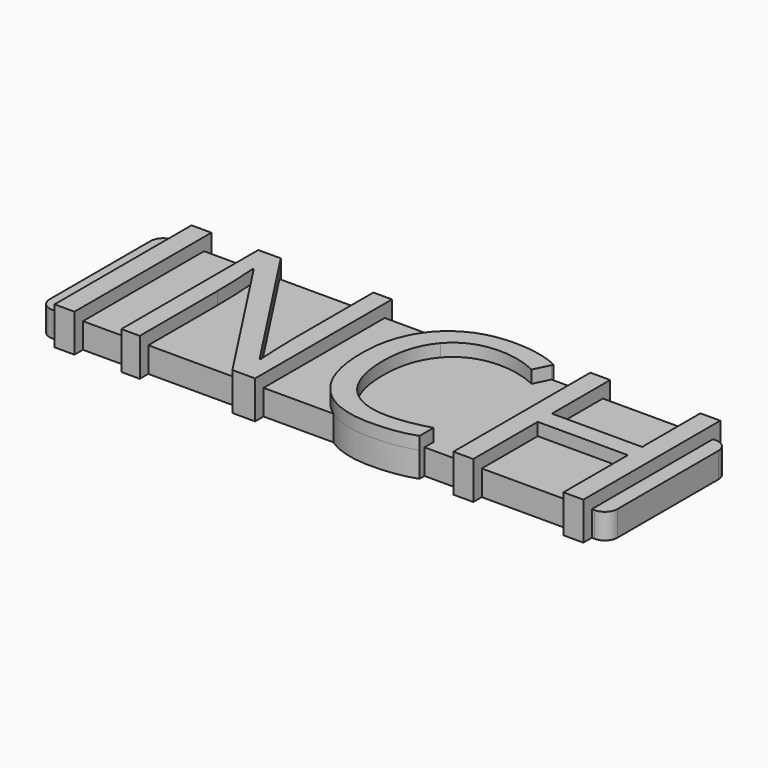
from build123d import *

# Parameters (mm, degrees)
F0_W          = 90
F0_H          = 24
F1_DEPTH      = 4
F2_R          = 2
F3_W          = 3.1525826242
F3_H          = 1.6790025727
F3_H_2        = 1.4474569563
F3_H_3        = 24
F3_W_2        = 2.9150999406
F3_W_3        = 2.9507223432
F4_DEPTH      = 2
F4_DEPTH_BACK = 4
F5_TEXT_SIZE  = 17.3611111111
F6_DEPTH      = 1.5


# Not quite as in the source:
# - a feature names something its author has since deleted; it is built from what else it names
# - Text() gives the source's letters only with a copy of the font that has no kerning and outlines rounded to 1/6400 em; it was checked with that copy


with BuildPart() as f1:
    # F0 (on Top) → F1 (new body)
    with BuildSketch(Plane.XY):
        Rectangle(F0_W, F0_H)
    extrude(amount=F1_DEPTH)

    # F2
    f2_edges = [f1.edges().sort_by_distance(p)[0] for p in [
        (-45, -12, 2),
        (45, 12, 2),
        (-45, 12, 2),
        (45, -12, 2),
    ]]
    fillet(f2_edges, radius=F2_R)

    # F3 (on face) → F4 (join, two sides)
    with BuildSketch(Plane.XY.offset(4)) as f4_sk:
        Polygon((-9.4904017415, -12), (-14.1817618998, -12), (-13.0882643974, -13.6790025727), (-9.4904017415, -13.6790025727), align=None)
        with Locations((-39.6952305561, -12.8395012864)):
            Rectangle(F3_W, F3_H)
        with Locations((-39.6952305561, 12.7237284781)):
            Rectangle(F3_W, F3_H_2)
        with Locations((-39.6952305561, 0)):
            Rectangle(F3_W, F3_H_3)
        with BuildLine():
            Line((-30.6797941817, 12), (-30.6797941817, -12))
            Line((-30.6797941817, -12), (-27.764694241, -12))
            Line((-27.764694241, -12), (-27.764694241, 1.739560657))
            add(Edge.make_bspline(
                [(-28.0615475955, 9.083712646), (-27.764694241, 5.076192361), (-27.764694241, 1.739560657)],
                knots=[0, 0, 0, 1, 1, 1], degree=2))
            Line((-28.0615475955, 9.083712646), (-27.9131209183, 9.083712646))
            Line((-27.9131209183, 9.083712646), (-14.1817618998, -12))
            Line((-14.1817618998, -12), (-9.4904017415, -12))
            Line((-9.4904017415, -12), (-9.4904017415, 12))
            Line((-9.4904017415, 12), (-12.4411240847, 12))
            Line((-12.4411240847, 12), (-12.4411240847, -2.1195329507))
            add(Edge.make_bspline(
                [(-12.3461310113, -6.0083118939), (-12.4767464872, -3.2891351672), (-12.4411240847, -2.1195329507)],
                knots=[0, 0, 0, 1, 1, 1], degree=2))
            add(Edge.make_bspline(
                [(-12.1798931328, -9.2262022561), (-12.2155155353, -8.7274886206), (-12.3461310113, -6.0083118939)],
                knots=[0, 0, 0, 1, 1, 1], degree=2))
            Line((-12.1798931328, -9.2262022561), (-12.32831981, -9.2262022561))
            Line((-12.32831981, -9.2262022561), (-26.17342843, 12))
            Line((-26.17342843, 12), (-30.6797941817, 12))
        make_face()
        with Locations((-29.2222442114, -12.8395012864)):
            Rectangle(F3_W_2, F3_H)
        Polygon((-30.6797941817, 13.4474569563), (-30.6797941817, 12), (-26.17342843, 12), (-27.1175539284, 13.4474569563), align=None)
        with BuildLine():
            add(Edge.make_bspline(
                [(1.606614259, -12), (0.6265764366, -11.3195654305), (-0.1840490798, -10.4136156739)],
                knots=[0.7510731854, 0.7510731854, 0.7510731854, 1, 1, 1], degree=2))
            Line((1.606614259, -12), (16.0211755393, -12))
            Line((16.0211755393, -12), (16.0211755393, -10.2295665941))
            add(Edge.make_bspline(
                [(9.5438353453, -11.2507421334), (12.3817534138, -11.2507421334), (16.0211755393, -10.2295665941)],
                knots=[0, 0, 0, 1, 1, 1], degree=2))
            add(Edge.make_bspline(
                [(2.4282604393, -8.3445477934), (4.9247971502, -11.2507421334), (9.5438353453, -11.2507421334)],
                knots=[0, 0, 0, 1, 1, 1], degree=2))
            add(Edge.make_bspline(
                [(-0.0682762715, -0.1187413418), (-0.0682762715, -5.4383534534), (2.4282604393, -8.3445477934)],
                knots=[0, 0, 0, 1, 1, 1], degree=2))
            add(Edge.make_bspline(
                [(2.5202849792, 8.0358203048), (-0.0682762715, 5.0583811597), (-0.0682762715, -0.1187413418)],
                knots=[0, 0, 0, 1, 1, 1], degree=2))
            add(Edge.make_bspline(
                [(9.5794577479, 11.0132594498), (5.10884623, 11.0132594498), (2.5202849792, 8.0358203048)],
                knots=[0, 0, 0, 1, 1, 1], degree=2))
            add(Edge.make_bspline(
                [(15.7421333861, 9.5705521472), (12.660795567, 11.0132594498), (9.5794577479, 11.0132594498)],
                knots=[0, 0, 0, 1, 1, 1], degree=2))
            Line((15.7421333861, 9.5705521472), (16.9408741029, 12))
            Line((16.9408741029, 12), (2.4397877824, 12))
            add(Edge.make_bspline(
                [(-1.8731446665, 7.2669701168), (-0.3629370603, 10.3045467792), (2.4397877824, 12)],
                knots=[0, 0, 0, 0.9635200801, 0.9635200801, 0.9635200801], degree=2))
            add(Edge.make_bspline(
                [(-3.440530378, -0.0771818722), (-3.440530378, 4.1143874926), (-1.8731446665, 7.2669701168)],
                knots=[0, 0, 0, 1, 1, 1], degree=2))
            add(Edge.make_bspline(
                [(-0.1840490798, -10.4136156739), (-3.440530378, -6.7741935484), (-3.440530378, -0.0771818722)],
                knots=[0, 0, 0, 1, 1, 1], degree=2))
        make_face()
        with BuildLine():
            Line((16.0211755393, -12), (1.606614259, -12))
            add(Edge.make_bspline(
                [(9.0629329111, -14.0530377993), (4.5636284737, -14.0530377993), (1.606614259, -12)],
                knots=[0, 0, 0, 0.7510731854, 0.7510731854, 0.7510731854], degree=2))
            add(Edge.make_bspline(
                [(16.0211755393, -12.9903027904), (13.2010686721, -14.0530377993), (9.0629329111, -14.0530377993)],
                knots=[0, 0, 0, 1, 1, 1], degree=2))
            Line((16.0211755393, -12.9903027904), (16.0211755393, -12))
        make_face()
        with Locations((40.959825846, -12.8395012864)):
            Rectangle(F3_W, F3_H)
        with BuildLine():
            add(Edge.make_bspline(
                [(2.4397877824, 12), (2.5459019983, 12.064191706), (2.6538689887, 12.126459529)],
                knots=[0.9635200801, 0.9635200801, 0.9635200801, 1, 1, 1], degree=2))
            Line((2.4397877824, 12), (16.9408741029, 12))
            Line((16.9408741029, 12), (17.0779734811, 12.2778547398))
            add(Edge.make_bspline(
                [(9.6210172175, 13.833366317), (13.8838313873, 13.833366317), (17.0779734811, 12.2778547398)],
                knots=[0, 0, 0, 1, 1, 1], degree=2))
            add(Edge.make_bspline(
                [(2.6538689887, 12.126459529), (5.6134969325, 13.833366317), (9.6210172175, 13.833366317)],
                knots=[0, 0, 0, 1, 1, 1], degree=2))
        make_face()
        with Locations((-10.9657629131, 12.7237284781)):
            Rectangle(F3_W_3, F3_H_2)
        with Locations((23.516722739, -12.8395012864)):
            Rectangle(F3_W, F3_H)
        Polygon((21.9404314269, 12), (21.9404314269, -12), (25.0930140511, -12), (25.0930140511, -0.9143083317), (39.3835345339, -0.9143083317), (39.3835345339, -12), (42.5361171581, -12), (42.5361171581, 12), (39.3835345339, 12), (39.3835345339, 1.9057985355), (25.0930140511, 1.9057985355), (25.0930140511, 12), align=None)
        with Locations((40.959825846, 12.7237284781)):
            Rectangle(F3_W, F3_H_2)
        with Locations((23.516722739, 12.7237284781)):
            Rectangle(F3_W, F3_H_2)
    extrude(amount=F4_DEPTH)
    extrude(f4_sk.sketch, amount=-F4_DEPTH_BACK)

    # F5 (on face) → F6 (cut)
    with BuildSketch(Plane(origin=(0, 0, 0), x_dir=(1, 0, 0), z_dir=(0, 0, -1))):
        with Locations((-31.5199110243, -6.25)):
            Text('2.54 cm', F5_TEXT_SIZE, font='Open Sans', text_align=(TextAlign.LEFT, TextAlign.BOTTOM))
    extrude(amount=-F6_DEPTH, mode=Mode.SUBTRACT)


solid = f1.part
